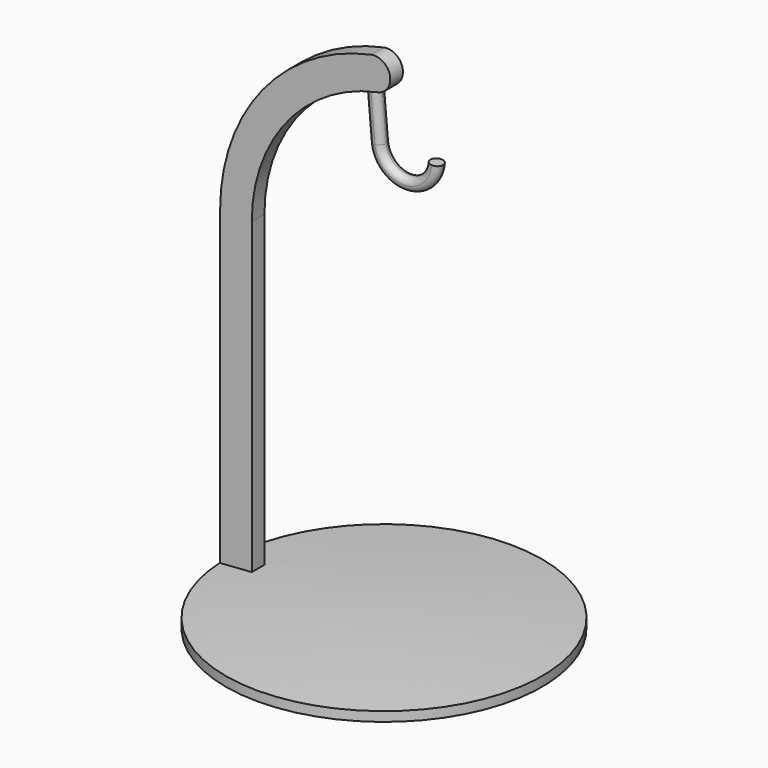
from build123d import *

# Parameters (mm, degrees)
F3_DEPTH = 3.175
F5_DEPTH = 2.54
F6_R     = 2.539


# Not quite as in the source:
# - a fillet or chamfer is up to 0.001 mm smaller than in the source, because OpenCascade refuses the exact size


with BuildPart() as f1:
    # F0 (on Right) → F1 (revolve)
    with BuildSketch(Plane.YZ):
        with BuildLine():
            Line((0, 6.35), (0, 0))
            Line((0, 0), (63.5, 0))
            Line((63.5, 0), (63.5, 3.81))
            ThreePointArc((63.5, 3.81), (31.7753898481, 5.714746203), (0, 6.35))
        make_face()
    revolve(axis=Axis((0, 0, 3.175), (0, 0, 1)))

    # F2 (on Front) → F3 (join, symmetric)
    with BuildSketch(Plane.XZ):
        with BuildLine():
            Line((-63.246, 0), (-50.546, 0))
            Line((-50.546, 0), (-50.546, 128.6024183169))
            ThreePointArc((-50.546, 128.6024183169), (-36.3147984428, 168.6628164677), (0, 190.7670697195))
            ThreePointArc((0, 190.7670697195), (4.9210651403, 198.2789348597), (-2.5908, 203.2))
            ThreePointArc((-2.5908, 203.2), (-46.1685581314, 176.6748960979), (-63.246, 128.6024183169))
            Line((-63.246, 128.6024183169), (-63.246, 0))
        make_face()
    extrude(amount=F3_DEPTH, both=True)

    # F4 (on Front) → F5 (join, symmetric)
    with BuildSketch(Plane.XZ):
        with BuildLine():
            Line((0.9183558658, 171.6801895282), (-1.2954, 196.9835348597))
            Line((-1.2954, 196.9835348597), (-6.3496308803, 196.4671948838))
            Line((-6.3496308803, 196.4671948838), (-4.1423132005, 171.2374383551))
            ThreePointArc((-4.1423132005, 171.2374383551), (9.8943909909, 158.4855183155), (23.7102105401, 171.4764251136))
            Line((23.7102105401, 171.4764251136), (18.6384196387, 171.7741938758))
            ThreePointArc((18.6384196387, 171.7741938758), (9.8216872219, 163.5651291728), (0.9183558658, 171.6801895282))
        make_face()
    extrude(amount=F5_DEPTH, both=True)

    # F6 (radius 2.54 in the source; OpenCascade refuses exactly that, so slightly less here)
    f6_edges = [f1.edges().sort_by_distance(p)[0] for p in [
        (0.090338, -2.54, 181.144481),
        (0.090338, 2.54, 181.144481),
        (9.821687, -2.54, 163.565129),
        (9.894391, -2.54, 158.485518),
        (-4.932181, -2.54, 180.265666),
        (9.894391, 2.54, 158.485518),
        (-4.932181, 2.54, 180.265666),
        (9.821687, 2.54, 163.565129),
    ]]
    fillet(f6_edges, radius=F6_R)


solid = f1.part
